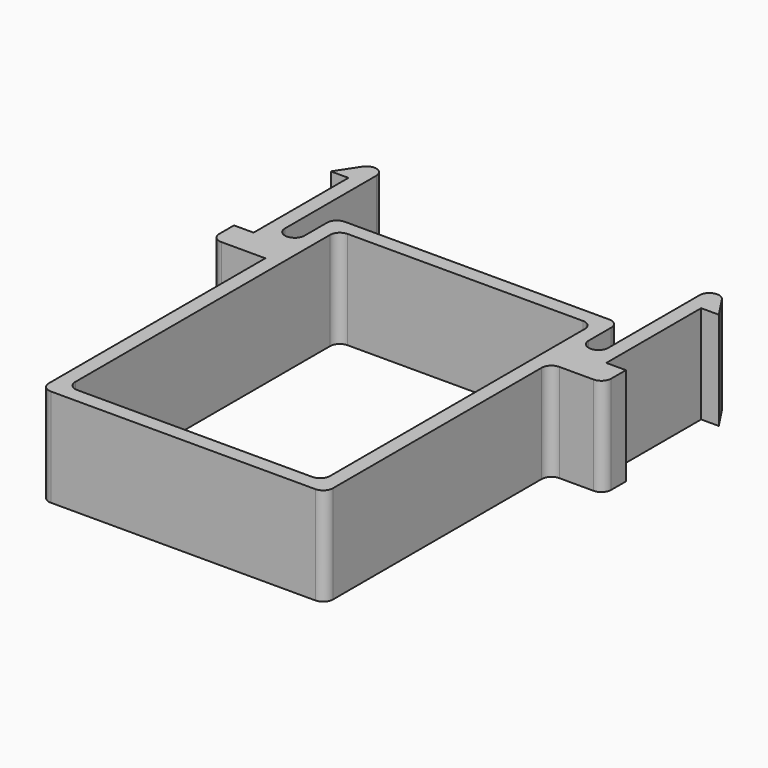
from build123d import *

# Parameters (mm, degrees)
F0_W     = 2
F0_H     = 4
F0_H_2   = 2.8740456328
F1_DEPTH = 10
F2_R     = 0.99999


# Not quite as in the source:
# - a fillet or chamfer is up to 0.001 mm smaller than in the source, because OpenCascade refuses the exact size


with BuildPart() as f1:
    # F0 (on Top) → F1 (new body)
    with BuildSketch(Plane.XY):
        Polygon((14.5, 18.75), (-14.5, 18.75), (-14.5, 13.8759543672), (-14.5, 9.8759543672), (-14.5, -18.75), (14.5, -18.75), (14.5, 9.8759543672), (14.5, 13.8759543672), align=None)
        Polygon((-13, 4.7144976147), (-13, 17.25), (13, 17.25), (13, 4.7144976147), (13, -2.2855023853), (13, -17.25), (-13, -17.25), (-13, -2.2855023853), align=None, mode=Mode.SUBTRACT)
        with Locations((-15.5, 11.8759543672)):
            Rectangle(F0_W, F0_H)
        Polygon((-16.5, 9.8759543672), (-16.5, 13.8759543672), (-16.5, 29.8609879265), (-19.8, 24.85), (-18, 24.85), (-18, 12.75), (-18, 9.8759543672), align=None)
        with Locations((15.5, 11.8759543672)):
            Rectangle(F0_W, F0_H)
        Polygon((16.5, 29.8609879265), (16.5, 13.8759543672), (16.5, 9.8759543672), (18, 9.8759543672), (18, 12.75), (18, 24.85), (19.8, 24.85), align=None)
        with Locations((-19, 11.3129771836)):
            Rectangle(F0_W, F0_H_2)
        with Locations((19, 11.3129771836)):
            Rectangle(F0_W, F0_H_2)
    extrude(amount=F1_DEPTH)

    # F2 (radius 1 in the source; OpenCascade refuses exactly that, so slightly less here)
    f2_edges = [f1.edges().sort_by_distance(p)[0] for p in [
        (-14.5, 18.75, 5),
        (-20, 9.875954, 5),
        (14.5, 18.75, 5),
        (20, 9.875954, 5),
        (-13, 17.25, 5),
        (14.5, 9.875954, 5),
        (14.5, -18.75, 5),
        (-14.5, -18.75, 5),
        (-13, -17.25, 5),
        (13, 17.25, 5),
        (13, -17.25, 5),
        (-14.5, 13.875954, 5),
        (16.5, 13.875954, 5),
        (-16.5, 13.875954, 5),
        (14.5, 13.875954, 5),
        (-16.5, 29.860988, 5),
        (16.5, 29.860988, 5),
    ]]
    fillet(f2_edges, radius=F2_R)


solid = f1.part
